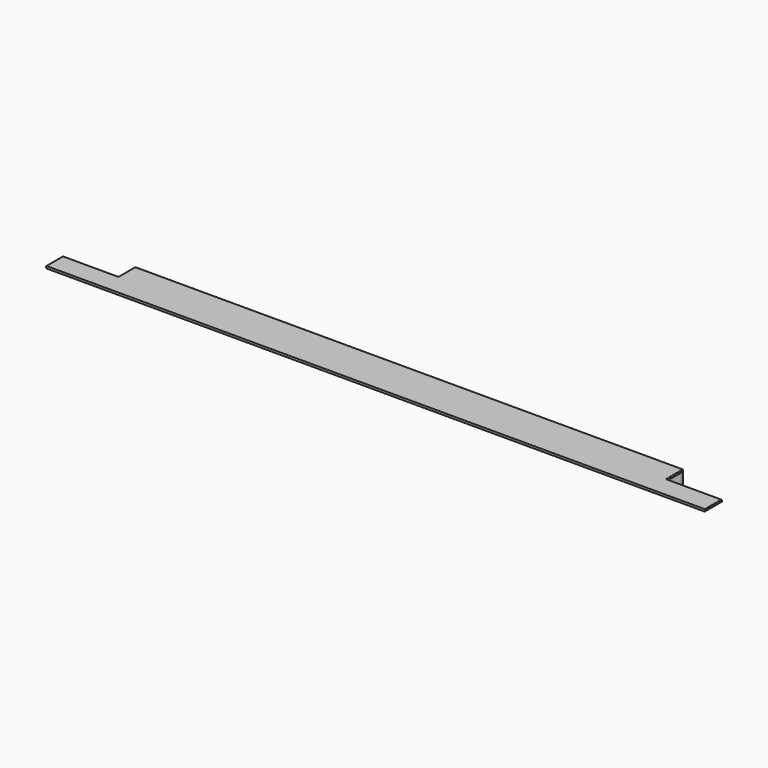
from build123d import *

# Parameters (mm, degrees)
F0_W           = 51.9615262747
F0_H           = 27.063280344
F1_DEPTH       = 38
F2_DEPTH       = 2
F3_DEPTH       = 594
F4_W           = 19
F4_H           = 2
F5_DEPTH       = 50
F6_W           = 19
F6_H           = 2
F7_DEPTH       = 50
F8_W           = 494
F8_H           = 9.5
F9_DEPTH       = 10
F10_DEPTH      = 7.5
F11_T1_DEPTH   = 10.9980686292
F11_T3_DEPTH   = 17
F11_T5_DEPTH   = 11.2524146128
F11_T7_DEPTH   = 21.5048292256
F11_T9_DEPTH   = 51.2524146128
F11_T11_DEPTH  = 492.9980686292
F11_T13_DEPTH  = 2.7514489274
F11_T15_DEPTH  = 18.4990343146
F11_T17_DEPTH  = 51.2524146128
F11_S21_W      = 0.5515022539
F11_S21_H      = 0.5515022539
F11_T22_DEPTH  = 0.551502254
F11_S27_W      = 0.5515022539
F11_S27_H      = 0.5515022539
F11_T28_DEPTH  = 0.551502254
F11_S33_W      = 0.5515022539
F11_S33_H      = 0.5515022539
F11_T34_DEPTH  = 0.551502254
F11_S39_W      = 0.5515022539
F11_S39_H      = 0.5515022539
F11_T40_DEPTH  = 0.551502254
F11_T47_DEPTH  = 51.2524146128
F11_T51_DEPTH  = 18.2524146128
F11_T58_DEPTH  = 18.2524146128
F11_T62_DEPTH  = 11.2524146128
F11_T69_DEPTH  = 18.2524146128
F11_T73_DEPTH  = 11.2524146128
F11_T80_DEPTH  = 19.7514489274
F11_T84_DEPTH  = 51.2524146128
F11_T91_DEPTH  = 18.2524146128
F11_T95_DEPTH  = 51.2524146128
F11_T102_DEPTH = 19.7514489274
F11_T106_DEPTH = 51.2524146128


# Not quite as in the source:
# - a fillet or chamfer that OpenCascade refuses, or shapes differently, is made with other operations: its cross-section is extruded or revolved along the edge and cut away or added
# - a feature names something its author has since deleted; it is built from what else it names


with BuildPart() as f1:
    # F0 (on Front) → F1 (new body)
    with BuildSketch(Plane.XZ):
        with Locations((-25.9807631373, 13.531640172)):
            Rectangle(F0_W, F0_H)
    extrude(amount=-F1_DEPTH)

    # F2 (intersect): a face of the model
    f2_faces = [f1.faces().sort_by_distance(p)[0] for p in [
        (-25.9807631373, 19, 0),
    ]]
    extrude(f2_faces, amount=-F2_DEPTH, mode=Mode.INTERSECT)

    # F3 (add): a face of the model
    f3_faces = [f1.faces().sort_by_distance(p)[0] for p in [
        (0, 19, 1),
    ]]
    extrude(f3_faces, amount=-F3_DEPTH)

    # F4 (on face) → F5 (cut)
    with BuildSketch(Plane.YZ):
        with Locations((28.5, 1)):
            Rectangle(F4_W, F4_H)
    extrude(amount=-F5_DEPTH, mode=Mode.SUBTRACT)

    # F6 (on face) → F7 (cut)
    with BuildSketch(Plane(origin=(-594, 0, 0), x_dir=(0, -1, 0), z_dir=(-1, 0, 0))):
        with Locations((-28.5, 1)):
            Rectangle(F6_W, F6_H)
    extrude(amount=-F7_DEPTH, mode=Mode.SUBTRACT)

    # F8 (on face) → F9 (join)
    with BuildSketch(Plane(origin=(0, 0, 0), x_dir=(1, 0, 0), z_dir=(0, 0, -1))):
        with Locations((-297, -33.25)):
            Rectangle(F8_W, F8_H)
    extrude(amount=F9_DEPTH)

    # F10 (cut): a face of the model
    f10_faces = [f1.faces().sort_by_distance(p)[0] for p in [
        (-297, 28.5, -5),
    ]]
    extrude(f10_faces, amount=-F10_DEPTH, mode=Mode.SUBTRACT)

    # F11: fillet of radius 0.5 on 21 edges, made by hand

    # F11_s2 → F11_t1 (cut)
    with BuildSketch(Plane.XY.offset(-9.4990343146)):
        with BuildLine():
            ThreePointArc((-543.4990343146, 38.0004), (-543.8535533906, 37.8535533906), (-544.0004, 37.4990343146))
            Line((-544.0004, 37.4990343146), (-544.0505365685, 37.4990343146))
            ThreePointArc((-544.0505365685, 37.4990343146), (-544.0501365685, 37.7495171573), (-544.0501365685, 38))
            Line((-544.0501365685, 38), (-544, 38.0501365685))
            ThreePointArc((-544, 38.0501365685), (-543.7495171573, 38.0501365685), (-543.4990343146, 38.0505365685))
            Line((-543.4990343146, 38.0505365685), (-543.4990343146, 38.0004))
        make_face()
        with BuildLine():
            ThreePointArc((-49.9996, 37.4990343146), (-50.1464466094, 37.8535533906), (-50.5009656854, 38.0004))
            Line((-50.5009656854, 38.0004), (-50.5009656854, 38.0505365685))
            ThreePointArc((-50.5009656854, 38.0505365685), (-50.2504828427, 38.0501365685), (-50, 38.0501365685))
            Line((-50, 38.0501365685), (-49.9498634315, 38))
            ThreePointArc((-49.9498634315, 38), (-49.9498634315, 37.7495171573), (-49.9494634315, 37.4990343146))
            Line((-49.9494634315, 37.4990343146), (-49.9996, 37.4990343146))
        make_face()
    extrude(amount=F11_T1_DEPTH, mode=Mode.SUBTRACT)

    # F11_s4 → F11_t3 (cut)
    with BuildSketch(Plane.XZ.offset(-36)):
        with BuildLine():
            ThreePointArc((-543.4990343146, -0.0004), (-543.8535533906, 0.1464466094), (-544.0004, 0.5009656854))
            Line((-544.0004, 0.5009656854), (-544.0505365685, 0.5009656854))
            ThreePointArc((-544.0505365685, 0.5009656854), (-544.0501365685, 0.2504828427), (-544.0501365685, 0))
            Line((-544.0501365685, 0), (-544, -0.0501365685))
            ThreePointArc((-544, -0.0501365685), (-543.7495171573, -0.0501365685), (-543.4990343146, -0.0505365685))
            Line((-543.4990343146, -0.0505365685), (-543.4990343146, -0.0004))
        make_face()
        with BuildLine():
            ThreePointArc((-50.5009656854, -0.0004), (-50.1464466094, 0.1464466094), (-49.9996, 0.5009656854))
            Line((-49.9996, 0.5009656854), (-49.9494634315, 0.5009656854))
            ThreePointArc((-49.9494634315, 0.5009656854), (-49.9498634315, 0.2504828427), (-49.9498634315, 0))
            Line((-49.9498634315, 0), (-50, -0.0501365685))
            ThreePointArc((-50, -0.0501365685), (-50.2504828427, -0.0501365685), (-50.5009656854, -0.0505365685))
            Line((-50.5009656854, -0.0505365685), (-50.5009656854, -0.0004))
        make_face()
    extrude(amount=F11_T3_DEPTH, mode=Mode.SUBTRACT)

    # F11_s6 → F11_t5 (cut)
    with BuildSketch(Plane.XY.offset(-11.2524146128)):
        with BuildLine():
            ThreePointArc((-543.4990343146, 35.9996), (-543.8535533906, 36.1464466094), (-544.0004, 36.5009656854))
            Line((-544.0004, 36.5009656854), (-544.0505365685, 36.5009656854))
            ThreePointArc((-544.0505365685, 36.5009656854), (-544.0501365685, 36.2504828427), (-544.0501365685, 36))
            Line((-544.0501365685, 36), (-544, 35.9498634315))
            ThreePointArc((-544, 35.9498634315), (-543.7495171573, 35.9498634315), (-543.4990343146, 35.9494634315))
            Line((-543.4990343146, 35.9494634315), (-543.4990343146, 35.9996))
        make_face()
        with BuildLine():
            ThreePointArc((-49.9996, 36.5009656854), (-50.1464466094, 36.1464466094), (-50.5009656854, 35.9996))
            Line((-50.5009656854, 35.9996), (-50.5009656854, 35.9494634315))
            ThreePointArc((-50.5009656854, 35.9494634315), (-50.2504828427, 35.9498634315), (-50, 35.9498634315))
            Line((-50, 35.9498634315), (-49.9498634315, 36))
            ThreePointArc((-49.9498634315, 36), (-49.9498634315, 36.2504828427), (-49.9494634315, 36.5009656854))
            Line((-49.9494634315, 36.5009656854), (-49.9996, 36.5009656854))
        make_face()
    extrude(amount=F11_T5_DEPTH, mode=Mode.SUBTRACT)

    # F11_s8 → F11_t7 (cut)
    with BuildSketch(Plane.XZ.offset(-20.2524146128)):
        with BuildLine():
            ThreePointArc((-593.4990343146, -0.0004), (-593.8535533906, 0.1464466094), (-594.0004, 0.5009656854))
            Line((-594.0004, 0.5009656854), (-594.0505365685, 0.5009656854))
            ThreePointArc((-594.0505365685, 0.5009656854), (-594.0501365685, 0.2504828427), (-594.0501365685, 0))
            Line((-594.0501365685, 0), (-594, -0.0501365685))
            ThreePointArc((-594, -0.0501365685), (-593.7495171573, -0.0501365685), (-593.4990343146, -0.0505365685))
            Line((-593.4990343146, -0.0505365685), (-593.4990343146, -0.0004))
        make_face()
        with BuildLine():
            ThreePointArc((0.0004, 0.5009656854), (-0.1464466094, 0.1464466094), (-0.5009656854, -0.0004))
            Line((-0.5009656854, -0.0004), (-0.5009656854, -0.0505365685))
            ThreePointArc((-0.5009656854, -0.0505365685), (-0.2504828427, -0.0501365685), (0, -0.0501365685))
            Line((0, -0.0501365685), (0.0501365685, 0))
            ThreePointArc((0.0501365685, 0), (0.0501365685, 0.2504828427), (0.0505365685, 0.5009656854))
            Line((0.0505365685, 0.5009656854), (0.0004, 0.5009656854))
        make_face()
        with BuildLine():
            ThreePointArc((0.0004, 1.4990343146), (-0.1464466094, 1.8535533906), (-0.5009656854, 2.0004))
            Line((-0.5009656854, 2.0004), (-0.5009656854, 2.0505365685))
            ThreePointArc((-0.5009656854, 2.0505365685), (-0.2504828427, 2.0501365685), (0, 2.0501365685))
            Line((0, 2.0501365685), (0.0501365685, 2))
            ThreePointArc((0.0501365685, 2), (0.0501365685, 1.7495171573), (0.0505365685, 1.4990343146))
            Line((0.0505365685, 1.4990343146), (0.0004, 1.4990343146))
        make_face()
        with BuildLine():
            ThreePointArc((-594.0004, 1.4990343146), (-593.8535533906, 1.8535533906), (-593.4990343146, 2.0004))
            Line((-593.4990343146, 2.0004), (-593.4990343146, 2.0505365685))
            ThreePointArc((-593.4990343146, 2.0505365685), (-593.7495171573, 2.0501365685), (-594, 2.0501365685))
            Line((-594, 2.0501365685), (-594.0501365685, 2))
            ThreePointArc((-594.0501365685, 2), (-594.0501365685, 1.7495171573), (-594.0505365685, 1.4990343146))
            Line((-594.0505365685, 1.4990343146), (-594.0004, 1.4990343146))
        make_face()
    extrude(amount=F11_T7_DEPTH, mode=Mode.SUBTRACT)

    # F11_s10 → F11_t9 (cut)
    with BuildSketch(Plane.YZ.offset(-595.2524146128)):
        with BuildLine():
            ThreePointArc((18.4990343146, -0.0004), (18.8535533906, 0.1464466094), (19.0004, 0.5009656854))
            Line((19.0004, 0.5009656854), (19.0505365685, 0.5009656854))
            ThreePointArc((19.0505365685, 0.5009656854), (19.0501365685, 0.2504828427), (19.0501365685, 0))
            Line((19.0501365685, 0), (19, -0.0501365685))
            ThreePointArc((19, -0.0501365685), (18.7495171573, -0.0501365685), (18.4990343146, -0.0505365685))
            Line((18.4990343146, -0.0505365685), (18.4990343146, -0.0004))
        make_face()
        with BuildLine():
            ThreePointArc((19.0004, 1.4990343146), (18.8535533906, 1.8535533906), (18.4990343146, 2.0004))
            Line((18.4990343146, 2.0004), (18.4990343146, 2.0505365685))
            ThreePointArc((18.4990343146, 2.0505365685), (18.7495171573, 2.0501365685), (19, 2.0501365685))
            Line((19, 2.0501365685), (19.0501365685, 2))
            ThreePointArc((19.0501365685, 2), (19.0501365685, 1.7495171573), (19.0505365685, 1.4990343146))
            Line((19.0505365685, 1.4990343146), (19.0004, 1.4990343146))
        make_face()
    extrude(amount=F11_T9_DEPTH, mode=Mode.SUBTRACT)

    # F11_s12 → F11_t11 (cut)
    with BuildSketch(Plane.YZ.offset(-543.4990343146)):
        with BuildLine():
            ThreePointArc((37.4990343146, -10.0004), (37.8535533906, -9.8535533906), (38.0004, -9.4990343146))
            Line((38.0004, -9.4990343146), (38.0505365685, -9.4990343146))
            ThreePointArc((38.0505365685, -9.4990343146), (38.0501365685, -9.7495171573), (38.0501365685, -10))
            Line((38.0501365685, -10), (38, -10.0501365685))
            ThreePointArc((38, -10.0501365685), (37.7495171573, -10.0501365685), (37.4990343146, -10.0505365685))
            Line((37.4990343146, -10.0505365685), (37.4990343146, -10.0004))
        make_face()
        with BuildLine():
            ThreePointArc((38.0004, 1.4990343146), (37.8535533906, 1.8535533906), (37.4990343146, 2.0004))
            Line((37.4990343146, 2.0004), (37.4990343146, 2.0505365685))
            ThreePointArc((37.4990343146, 2.0505365685), (37.7495171573, 2.0501365685), (38, 2.0501365685))
            Line((38, 2.0501365685), (38.0501365685, 2))
            ThreePointArc((38.0501365685, 2), (38.0501365685, 1.7495171573), (38.0505365685, 1.4990343146))
            Line((38.0505365685, 1.4990343146), (38.0004, 1.4990343146))
        make_face()
    extrude(amount=F11_T11_DEPTH, mode=Mode.SUBTRACT)

    # F11_s14 → F11_t13 (cut)
    with BuildSketch(Plane.XZ.offset(-37.4990343146)):
        with BuildLine():
            ThreePointArc((-543.4990343146, -10.0004), (-543.8535533906, -9.8535533906), (-544.0004, -9.4990343146))
            Line((-544.0004, -9.4990343146), (-544.0505365685, -9.4990343146))
            ThreePointArc((-544.0505365685, -9.4990343146), (-544.0501365685, -9.7495171573), (-544.0501365685, -10))
            Line((-544.0501365685, -10), (-544, -10.0501365685))
            ThreePointArc((-544, -10.0501365685), (-543.7495171573, -10.0501365685), (-543.4990343146, -10.0505365685))
            Line((-543.4990343146, -10.0505365685), (-543.4990343146, -10.0004))
        make_face()
        with BuildLine():
            ThreePointArc((-49.9996, -9.4990343146), (-50.1464466094, -9.8535533906), (-50.5009656854, -10.0004))
            Line((-50.5009656854, -10.0004), (-50.5009656854, -10.0505365685))
            ThreePointArc((-50.5009656854, -10.0505365685), (-50.2504828427, -10.0501365685), (-50, -10.0501365685))
            Line((-50, -10.0501365685), (-49.9498634315, -10))
            ThreePointArc((-49.9498634315, -10), (-49.9498634315, -9.7495171573), (-49.9494634315, -9.4990343146))
            Line((-49.9494634315, -9.4990343146), (-49.9996, -9.4990343146))
        make_face()
    extrude(amount=F11_T13_DEPTH, mode=Mode.SUBTRACT)

    # F11_s16 → F11_t15 (cut)
    with BuildSketch(Plane.XZ.offset(-37.4990343146)):
        with BuildLine():
            ThreePointArc((-49.9996, 1.4990343146), (-50.1464466094, 1.8535533906), (-50.5009656854, 2.0004))
            Line((-50.5009656854, 2.0004), (-50.5009656854, 2.0505365685))
            ThreePointArc((-50.5009656854, 2.0505365685), (-50.2504828427, 2.0501365685), (-50, 2.0501365685))
            Line((-50, 2.0501365685), (-49.9498634315, 2))
            ThreePointArc((-49.9498634315, 2), (-49.9498634315, 1.7495171573), (-49.9494634315, 1.4990343146))
            Line((-49.9494634315, 1.4990343146), (-49.9996, 1.4990343146))
        make_face()
        with BuildLine():
            ThreePointArc((-544.0004, 1.4990343146), (-543.8535533906, 1.8535533906), (-543.4990343146, 2.0004))
            Line((-543.4990343146, 2.0004), (-543.4990343146, 2.0505365685))
            ThreePointArc((-543.4990343146, 2.0505365685), (-543.7495171573, 2.0501365685), (-544, 2.0501365685))
            Line((-544, 2.0501365685), (-544.0501365685, 2))
            ThreePointArc((-544.0501365685, 2), (-544.0501365685, 1.7495171573), (-544.0505365685, 1.4990343146))
            Line((-544.0505365685, 1.4990343146), (-544.0004, 1.4990343146))
        make_face()
    extrude(amount=F11_T15_DEPTH, mode=Mode.SUBTRACT)

    # F11_s18 → F11_t17 (cut)
    with BuildSketch(Plane.YZ.offset(-50)):
        with BuildLine():
            ThreePointArc((19.0004, 1.4990343146), (18.8535533906, 1.8535533906), (18.4990343146, 2.0004))
            Line((18.4990343146, 2.0004), (18.4990343146, 2.0505365685))
            ThreePointArc((18.4990343146, 2.0505365685), (18.7495171573, 2.0501365685), (19, 2.0501365685))
            Line((19, 2.0501365685), (19.0501365685, 2))
            ThreePointArc((19.0501365685, 2), (19.0501365685, 1.7495171573), (19.0505365685, 1.4990343146))
            Line((19.0505365685, 1.4990343146), (19.0004, 1.4990343146))
        make_face()
        with BuildLine():
            ThreePointArc((18.4990343146, -0.0004), (18.8535533906, 0.1464466094), (19.0004, 0.5009656854))
            Line((19.0004, 0.5009656854), (19.0505365685, 0.5009656854))
            ThreePointArc((19.0505365685, 0.5009656854), (19.0501365685, 0.2504828427), (19.0501365685, 0))
            Line((19.0501365685, 0), (19, -0.0501365685))
            ThreePointArc((19, -0.0501365685), (18.7495171573, -0.0501365685), (18.4990343146, -0.0505365685))
            Line((18.4990343146, -0.0505365685), (18.4990343146, -0.0004))
        make_face()
    extrude(amount=F11_T17_DEPTH, mode=Mode.SUBTRACT)


with BuildPart() as f11_tool20:
    # F11_s21 → F11_t22 (new body)
    with BuildSketch(Plane.XY.offset(-9.4990343146)):
        with Locations((-543.7747854415, 37.7747854416)):
            Rectangle(F11_S21_W, F11_S21_H)
    extrude(amount=-F11_T22_DEPTH)

    # F11_s23 → F11_t24 (revolve, cut)
    with BuildSketch(Plane(origin=(-543.4990343146, 37.4990343146, -9.4990343146), x_dir=(0.7071067812, -0.7071067812, 0), z_dir=(0.7071067812, 0.7071067812, 0))):
        with BuildLine():
            ThreePointArc((0, -0.5013656854), (0.5013656854, 0), (0, 0.5013656854))
            Line((0, 0.5013656854), (0, -0.5013656854))
        make_face()
    revolve(axis=Axis((-543.4990343146, 37.4990343146, -9.4990343146), (0, 0, -1)), mode=Mode.SUBTRACT)


with BuildPart() as f1_1:
    add(f1.part)

    # F11_t19: cut F11_tool20
    add(f11_tool20.part, mode=Mode.SUBTRACT)


with BuildPart() as f11_tool26:
    # F11_s27 → F11_t28 (new body)
    with BuildSketch(Plane.XY.offset(1.4990343146)):
        with Locations((-543.7747854415, 37.7747854416)):
            Rectangle(F11_S27_W, F11_S27_H)
    extrude(amount=F11_T28_DEPTH)

    # F11_s29 → F11_t30 (revolve, cut)
    with BuildSketch(Plane(origin=(-543.4990343146, 37.4990343146, 1.4990343146), x_dir=(0.7071067812, -0.7071067812, 0), z_dir=(-0.7071067812, -0.7071067812, 0))):
        with BuildLine():
            ThreePointArc((0, -0.5013656854), (0.5013656854, 0), (0, 0.5013656854))
            Line((0, 0.5013656854), (0, -0.5013656854))
        make_face()
    revolve(axis=Axis((-543.4990343146, 37.4990343146, 1.4990343146), (0, 0, 1)), mode=Mode.SUBTRACT)


with BuildPart() as f1_2:
    add(f1_1.part)

    # F11_t25: cut F11_tool26
    add(f11_tool26.part, mode=Mode.SUBTRACT)


with BuildPart() as f11_tool32:
    # F11_s33 → F11_t34 (new body)
    with BuildSketch(Plane.YZ.offset(-50.5009656854)):
        with Locations((37.7747854416, -9.7747854415)):
            Rectangle(F11_S33_W, F11_S33_H)
    extrude(amount=F11_T34_DEPTH)

    # F11_s35 → F11_t36 (revolve, cut)
    with BuildSketch(Plane(origin=(-50.5009656854, 37.4990343146, -9.4990343146), x_dir=(0, -0.7071067812, 0.7071067812), z_dir=(0, 0.7071067812, 0.7071067812))):
        with BuildLine():
            ThreePointArc((0, -0.5013656854), (0.5013656854, 0), (0, 0.5013656854))
            Line((0, 0.5013656854), (0, -0.5013656854))
        make_face()
    revolve(axis=Axis((-50.5009656854, 37.4990343146, -9.4990343146), (1, 0, 0)), mode=Mode.SUBTRACT)


with BuildPart() as f1_3:
    add(f1_2.part)

    # F11_t31: cut F11_tool32
    add(f11_tool32.part, mode=Mode.SUBTRACT)


with BuildPart() as f11_tool38:
    # F11_s39 → F11_t40 (new body)
    with BuildSketch(Plane.YZ.offset(-50.5009656854)):
        with Locations((37.7747854416, 1.7747854416)):
            Rectangle(F11_S39_W, F11_S39_H)
    extrude(amount=F11_T40_DEPTH)

    # F11_s41 → F11_t42 (revolve, cut)
    with BuildSketch(Plane(origin=(-50.5009656854, 37.4990343146, 1.4990343146), x_dir=(0, -0.7071067812, -0.7071067812), z_dir=(0, -0.7071067812, 0.7071067812))):
        with BuildLine():
            ThreePointArc((0, -0.5013656854), (0.5013656854, 0), (0, 0.5013656854))
            Line((0, 0.5013656854), (0, -0.5013656854))
        make_face()
    revolve(axis=Axis((-50.5009656854, 37.4990343146, 1.4990343146), (1, 0, 0)), mode=Mode.SUBTRACT)


with BuildPart() as f1_4:
    add(f1_3.part)

    # F11_t37: cut F11_tool38
    add(f11_tool38.part, mode=Mode.SUBTRACT)


with BuildPart() as f11_tool45:
    # F11_s46 → F11_t47 (new body)
    with BuildSketch(Plane.YZ.offset(-594)):
        with BuildLine():
            ThreePointArc((18.4990343146, -0.0004), (18.8535533906, 0.1464466094), (19.0004, 0.5009656854))
            Line((19.0004, 0.5009656854), (19.0505365685, 0.5009656854))
            ThreePointArc((19.0505365685, 0.5009656854), (19.0501365685, 0.2504828427), (19.0501365685, 0))
            Line((19.0501365685, 0), (19, -0.0501365685))
            ThreePointArc((19, -0.0501365685), (18.7495171573, -0.0501365685), (18.4990343146, -0.0505365685))
            Line((18.4990343146, -0.0505365685), (18.4990343146, -0.0004))
        make_face()
    extrude(amount=F11_T47_DEPTH)

    split(bisect_by=Plane.YZ.offset(-544), keep=Keep.TOP)


with BuildPart() as f11_tool49:
    # F11_s50 → F11_t51 (new body)
    with BuildSketch(Plane.XZ.offset(-17.7475853872)):
        with BuildLine():
            ThreePointArc((-543.4990343146, -0.0004), (-543.8535533906, 0.1464466094), (-544.0004, 0.5009656854))
            Line((-544.0004, 0.5009656854), (-544.0505365685, 0.5009656854))
            ThreePointArc((-544.0505365685, 0.5009656854), (-544.0501365685, 0.2504828427), (-544.0501365685, 0))
            Line((-544.0501365685, 0), (-544, -0.0501365685))
            ThreePointArc((-544, -0.0501365685), (-543.7495171573, -0.0501365685), (-543.4990343146, -0.0505365685))
            Line((-543.4990343146, -0.0505365685), (-543.4990343146, -0.0004))
        make_face()
    extrude(amount=-F11_T51_DEPTH)

    split(bisect_by=Plane.XZ.offset(-19), keep=Keep.TOP)


with BuildPart() as f11_tool45_1:
    add(f11_tool45.part)

    # F11_t53: intersect F11_tool49
    add(f11_tool49.part, mode=Mode.INTERSECT)


with BuildPart() as f1_5:
    add(f1_4.part)

    # F11_t43: cut F11_tool45
    add(f11_tool45_1.part, mode=Mode.SUBTRACT)


with BuildPart() as f11_tool56:
    # F11_s57 → F11_t58 (new body)
    with BuildSketch(Plane.XZ.offset(-19)):
        with BuildLine():
            ThreePointArc((-543.4990343146, -0.0004), (-543.8535533906, 0.1464466094), (-544.0004, 0.5009656854))
            Line((-544.0004, 0.5009656854), (-544.0505365685, 0.5009656854))
            ThreePointArc((-544.0505365685, 0.5009656854), (-544.0501365685, 0.2504828427), (-544.0501365685, 0))
            Line((-544.0501365685, 0), (-544, -0.0501365685))
            ThreePointArc((-544, -0.0501365685), (-543.7495171573, -0.0501365685), (-543.4990343146, -0.0505365685))
            Line((-543.4990343146, -0.0505365685), (-543.4990343146, -0.0004))
        make_face()
    extrude(amount=-F11_T58_DEPTH)

    split(bisect_by=Plane.XZ.offset(-36), keep=Keep.BOTTOM)


with BuildPart() as f11_tool60:
    # F11_s61 → F11_t62 (new body)
    with BuildSketch(Plane.XY.offset(1.2524146128)):
        with BuildLine():
            ThreePointArc((-543.4990343146, 35.9996), (-543.8535533906, 36.1464466094), (-544.0004, 36.5009656854))
            Line((-544.0004, 36.5009656854), (-544.0505365685, 36.5009656854))
            ThreePointArc((-544.0505365685, 36.5009656854), (-544.0501365685, 36.2504828427), (-544.0501365685, 36))
            Line((-544.0501365685, 36), (-544, 35.9498634315))
            ThreePointArc((-544, 35.9498634315), (-543.7495171573, 35.9498634315), (-543.4990343146, 35.9494634315))
            Line((-543.4990343146, 35.9494634315), (-543.4990343146, 35.9996))
        make_face()
    extrude(amount=-F11_T62_DEPTH)

    split(bisect_by=Plane.XY, keep=Keep.TOP)


with BuildPart() as f11_tool56_1:
    add(f11_tool56.part)

    # F11_t64: intersect F11_tool60
    add(f11_tool60.part, mode=Mode.INTERSECT)


with BuildPart() as f1_6:
    add(f1_5.part)

    # F11_t54: cut F11_tool56
    add(f11_tool56_1.part, mode=Mode.SUBTRACT)


with BuildPart() as f11_tool67:
    # F11_s68 → F11_t69 (new body)
    with BuildSketch(Plane.XZ.offset(-37.2524146128)):
        with BuildLine():
            ThreePointArc((-50.5009656854, -0.0004), (-50.1464466094, 0.1464466094), (-49.9996, 0.5009656854))
            Line((-49.9996, 0.5009656854), (-49.9494634315, 0.5009656854))
            ThreePointArc((-49.9494634315, 0.5009656854), (-49.9498634315, 0.2504828427), (-49.9498634315, 0))
            Line((-49.9498634315, 0), (-50, -0.0501365685))
            ThreePointArc((-50, -0.0501365685), (-50.2504828427, -0.0501365685), (-50.5009656854, -0.0505365685))
            Line((-50.5009656854, -0.0505365685), (-50.5009656854, -0.0004))
        make_face()
    extrude(amount=F11_T69_DEPTH)

    split(bisect_by=Plane.XZ.offset(-36), keep=Keep.BOTTOM)


with BuildPart() as f11_tool71:
    # F11_s72 → F11_t73 (new body)
    with BuildSketch(Plane.XY.offset(1.2524146128)):
        with BuildLine():
            ThreePointArc((-49.9996, 36.5009656854), (-50.1464466094, 36.1464466094), (-50.5009656854, 35.9996))
            Line((-50.5009656854, 35.9996), (-50.5009656854, 35.9494634315))
            ThreePointArc((-50.5009656854, 35.9494634315), (-50.2504828427, 35.9498634315), (-50, 35.9498634315))
            Line((-50, 35.9498634315), (-49.9498634315, 36))
            ThreePointArc((-49.9498634315, 36), (-49.9498634315, 36.2504828427), (-49.9494634315, 36.5009656854))
            Line((-49.9494634315, 36.5009656854), (-49.9996, 36.5009656854))
        make_face()
    extrude(amount=-F11_T73_DEPTH)

    split(bisect_by=Plane.XY, keep=Keep.TOP)


with BuildPart() as f11_tool67_1:
    add(f11_tool67.part)

    # F11_t75: intersect F11_tool71
    add(f11_tool71.part, mode=Mode.INTERSECT)


with BuildPart() as f1_7:
    add(f1_6.part)

    # F11_t65: cut F11_tool67
    add(f11_tool67_1.part, mode=Mode.SUBTRACT)


with BuildPart() as f11_tool78:
    # F11_s79 → F11_t80 (new body)
    with BuildSketch(Plane.XZ.offset(-37.4990343146)):
        with BuildLine():
            ThreePointArc((-49.9996, 1.4990343146), (-50.1464466094, 1.8535533906), (-50.5009656854, 2.0004))
            Line((-50.5009656854, 2.0004), (-50.5009656854, 2.0505365685))
            ThreePointArc((-50.5009656854, 2.0505365685), (-50.2504828427, 2.0501365685), (-50, 2.0501365685))
            Line((-50, 2.0501365685), (-49.9498634315, 2))
            ThreePointArc((-49.9498634315, 2), (-49.9498634315, 1.7495171573), (-49.9494634315, 1.4990343146))
            Line((-49.9494634315, 1.4990343146), (-49.9996, 1.4990343146))
        make_face()
    extrude(amount=F11_T80_DEPTH)

    split(bisect_by=Plane.XZ.offset(-19), keep=Keep.TOP)


with BuildPart() as f11_tool82:
    # F11_s83 → F11_t84 (new body)
    with BuildSketch(Plane.YZ):
        with BuildLine():
            ThreePointArc((19.0004, 1.4990343146), (18.8535533906, 1.8535533906), (18.4990343146, 2.0004))
            Line((18.4990343146, 2.0004), (18.4990343146, 2.0505365685))
            ThreePointArc((18.4990343146, 2.0505365685), (18.7495171573, 2.0501365685), (19, 2.0501365685))
            Line((19, 2.0501365685), (19.0501365685, 2))
            ThreePointArc((19.0501365685, 2), (19.0501365685, 1.7495171573), (19.0505365685, 1.4990343146))
            Line((19.0505365685, 1.4990343146), (19.0004, 1.4990343146))
        make_face()
    extrude(amount=-F11_T84_DEPTH)

    split(bisect_by=Plane.YZ.offset(-50), keep=Keep.BOTTOM)


with BuildPart() as f11_tool78_1:
    add(f11_tool78.part)

    # F11_t86: intersect F11_tool82
    add(f11_tool82.part, mode=Mode.INTERSECT)


with BuildPart() as f1_8:
    add(f1_7.part)

    # F11_t76: cut F11_tool78
    add(f11_tool78_1.part, mode=Mode.SUBTRACT)


with BuildPart() as f11_tool89:
    # F11_s90 → F11_t91 (new body)
    with BuildSketch(Plane.XZ.offset(-36)):
        with BuildLine():
            ThreePointArc((-50.5009656854, -0.0004), (-50.1464466094, 0.1464466094), (-49.9996, 0.5009656854))
            Line((-49.9996, 0.5009656854), (-49.9494634315, 0.5009656854))
            ThreePointArc((-49.9494634315, 0.5009656854), (-49.9498634315, 0.2504828427), (-49.9498634315, 0))
            Line((-49.9498634315, 0), (-50, -0.0501365685))
            ThreePointArc((-50, -0.0501365685), (-50.2504828427, -0.0501365685), (-50.5009656854, -0.0505365685))
            Line((-50.5009656854, -0.0505365685), (-50.5009656854, -0.0004))
        make_face()
    extrude(amount=F11_T91_DEPTH)

    split(bisect_by=Plane.XZ.offset(-19), keep=Keep.TOP)


with BuildPart() as f11_tool93:
    # F11_s94 → F11_t95 (new body)
    with BuildSketch(Plane.YZ):
        with BuildLine():
            ThreePointArc((18.4990343146, -0.0004), (18.8535533906, 0.1464466094), (19.0004, 0.5009656854))
            Line((19.0004, 0.5009656854), (19.0505365685, 0.5009656854))
            ThreePointArc((19.0505365685, 0.5009656854), (19.0501365685, 0.2504828427), (19.0501365685, 0))
            Line((19.0501365685, 0), (19, -0.0501365685))
            ThreePointArc((19, -0.0501365685), (18.7495171573, -0.0501365685), (18.4990343146, -0.0505365685))
            Line((18.4990343146, -0.0505365685), (18.4990343146, -0.0004))
        make_face()
    extrude(amount=-F11_T95_DEPTH)

    split(bisect_by=Plane.YZ.offset(-50), keep=Keep.BOTTOM)


with BuildPart() as f11_tool89_1:
    add(f11_tool89.part)

    # F11_t97: intersect F11_tool93
    add(f11_tool93.part, mode=Mode.INTERSECT)


with BuildPart() as f1_9:
    add(f1_8.part)

    # F11_t87: cut F11_tool89
    add(f11_tool89_1.part, mode=Mode.SUBTRACT)


with BuildPart() as f11_tool100:
    # F11_s101 → F11_t102 (new body)
    with BuildSketch(Plane.XZ.offset(-17.7475853872)):
        with BuildLine():
            ThreePointArc((-544.0004, 1.4990343146), (-543.8535533906, 1.8535533906), (-543.4990343146, 2.0004))
            Line((-543.4990343146, 2.0004), (-543.4990343146, 2.0505365685))
            ThreePointArc((-543.4990343146, 2.0505365685), (-543.7495171573, 2.0501365685), (-544, 2.0501365685))
            Line((-544, 2.0501365685), (-544.0501365685, 2))
            ThreePointArc((-544.0501365685, 2), (-544.0501365685, 1.7495171573), (-544.0505365685, 1.4990343146))
            Line((-544.0505365685, 1.4990343146), (-544.0004, 1.4990343146))
        make_face()
    extrude(amount=-F11_T102_DEPTH)

    split(bisect_by=Plane.XZ.offset(-19), keep=Keep.TOP)


with BuildPart() as f11_tool104:
    # F11_s105 → F11_t106 (new body)
    with BuildSketch(Plane.YZ.offset(-594)):
        with BuildLine():
            ThreePointArc((19.0004, 1.4990343146), (18.8535533906, 1.8535533906), (18.4990343146, 2.0004))
            Line((18.4990343146, 2.0004), (18.4990343146, 2.0505365685))
            ThreePointArc((18.4990343146, 2.0505365685), (18.7495171573, 2.0501365685), (19, 2.0501365685))
            Line((19, 2.0501365685), (19.0501365685, 2))
            ThreePointArc((19.0501365685, 2), (19.0501365685, 1.7495171573), (19.0505365685, 1.4990343146))
            Line((19.0505365685, 1.4990343146), (19.0004, 1.4990343146))
        make_face()
    extrude(amount=F11_T106_DEPTH)

    split(bisect_by=Plane.YZ.offset(-544), keep=Keep.TOP)


with BuildPart() as f11_tool100_1:
    add(f11_tool100.part)

    # F11_t108: intersect F11_tool104
    add(f11_tool104.part, mode=Mode.INTERSECT)


with BuildPart() as f1_10:
    add(f1_9.part)

    # F11_t98: cut F11_tool100
    add(f11_tool100_1.part, mode=Mode.SUBTRACT)


solid = f1_10.part
